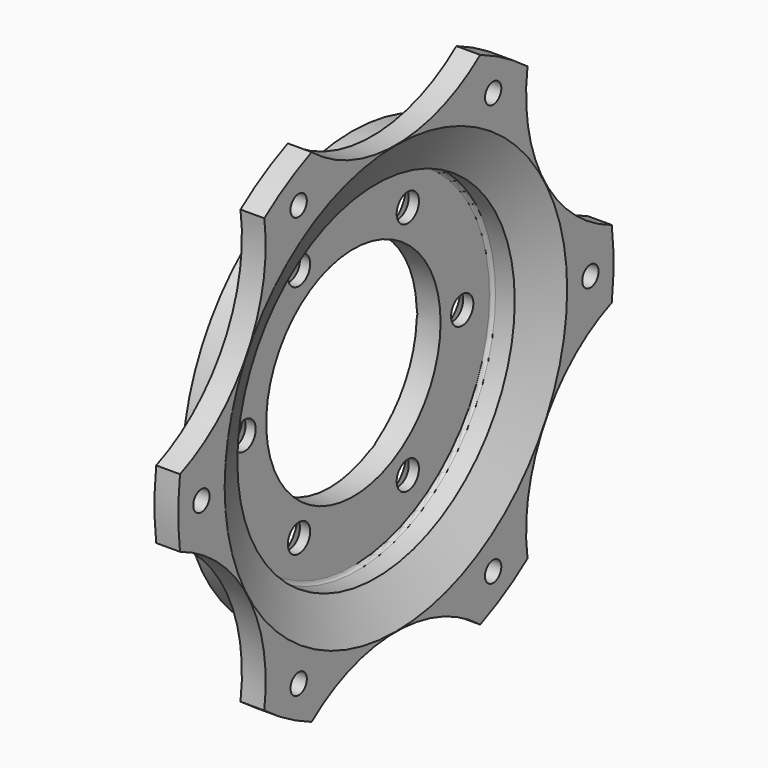
from build123d import *

# Parameters (mm, degrees)
F2_R     = 4.1
F3_DEPTH = 50
F4_R     = 3
F5_DEPTH = 50
F7_R     = 1
F8_R     = 50
F9_DEPTH = 50


# Not quite as in the source:
# - a fillet or chamfer that OpenCascade refuses, or shapes differently, is made with other operations: its cross-section is extruded or revolved along the edge and cut away or added
# - a feature names something its author has since deleted; it is built from what else it names


with BuildPart() as f1:
    # F0 (on Top) → F1 (revolve)
    with BuildSketch(Plane.XY):
        Polygon((-7, 49), (-7, 32.05), (0, 32.05), (0, 51), (6.6556592449, 51), (12.5, 62.9584203143), (12.5, 80), (5.5, 80), (5.5, 62.3), (-0.5, 62.3), align=None)
    revolve(axis=Axis((-3.5, 0, 0), (1, 0, 0)))

    # F2 (on Right) → F3 (cut, symmetric)
    with BuildSketch(Plane.YZ):
        with Locations((-40, 0)):
            Circle(F2_R)
        with Locations((-20, -34.6410161514)):
            Circle(F2_R)
        with Locations((20, -34.6410161514)):
            Circle(F2_R)
        with Locations((40, 0)):
            Circle(F2_R)
        with Locations((20, 34.6410161514)):
            Circle(F2_R)
        with Locations((-20, 34.6410161514)):
            Circle(F2_R)
    extrude(amount=F3_DEPTH, both=True, mode=Mode.SUBTRACT)

    # F4 (on face) → F5 (cut, symmetric)
    with BuildSketch(Plane(origin=(5.5, 0, 0), x_dir=(0, -1, 0), z_dir=(-1, 0, 0))):
        with Locations((35.75, 61.9208163706)):
            Circle(F4_R)
        with Locations((-35.75, 61.9208163706)):
            Circle(F4_R)
        with Locations((-71.5, 0)):
            Circle(F4_R)
        with Locations((-35.75, -61.9208163706)):
            Circle(F4_R)
        with Locations((35.75, -61.9208163706)):
            Circle(F4_R)
        with Locations((71.5, 0)):
            Circle(F4_R)
    extrude(amount=F5_DEPTH, both=True, mode=Mode.SUBTRACT)

    # F6: chamfer of 4 on 6 edges, made by hand

    # F6_s1 → F6_t2 (revolve, cut)
    with BuildSketch(Plane.XY.offset(34.6410161514)):
        Polygon((-7, 28.1), (-3, 24.1), (-7, 24.1), align=None)
    revolve(axis=Axis((-7, 20, 34.6410161514), (1, 0, 0)), mode=Mode.SUBTRACT)

    # F6_s3 → F6_t4 (revolve, cut)
    with BuildSketch(Plane.XY.offset(34.6410161514)):
        Polygon((-7, -11.9), (-3, -15.9), (-7, -15.9), align=None)
    revolve(axis=Axis((-7, -20, 34.6410161514), (1, 0, 0)), mode=Mode.SUBTRACT)

    # F6_s5 → F6_t6 (revolve, cut)
    with BuildSketch(Plane.XY):
        Polygon((-7, -31.9), (-3, -35.9), (-7, -35.9), align=None)
    revolve(axis=Axis((-7, -40, 0), (1, 0, 0)), mode=Mode.SUBTRACT)

    # F6_s7 → F6_t8 (revolve, cut)
    with BuildSketch(Plane.XY.offset(-34.6410161514)):
        Polygon((-7, -11.9), (-3, -15.9), (-7, -15.9), align=None)
    revolve(axis=Axis((-7, -20, -34.6410161514), (1, 0, 0)), mode=Mode.SUBTRACT)

    # F6_s9 → F6_t10 (revolve, cut)
    with BuildSketch(Plane.XY.offset(-34.6410161514)):
        Polygon((-7, 28.1), (-3, 24.1), (-7, 24.1), align=None)
    revolve(axis=Axis((-7, 20, -34.6410161514), (1, 0, 0)), mode=Mode.SUBTRACT)

    # F6_s11 → F6_t12 (revolve, cut)
    with BuildSketch(Plane.XY):
        Polygon((-7, 48.1), (-3, 44.1), (-7, 44.1), align=None)
    revolve(axis=Axis((-7, 40, 0), (1, 0, 0)), mode=Mode.SUBTRACT)

    # F7
    f7_edges = [f1.edges().sort_by_distance(p)[0] for p in [
        (0, -51, 0),
    ]]
    fillet(f7_edges, radius=F7_R)

    # F8 (on face) → F9 (cut, symmetric)
    with BuildSketch(Plane(origin=(5.5, 0, 0), x_dir=(0, -1, 0), z_dir=(-1, 0, 0))):
        with Locations((0, 113)):
            Circle(F8_R)
        with Locations((-97.8608706276, 56.5)):
            Circle(F8_R)
        with Locations((-97.8608706276, -56.5)):
            Circle(F8_R)
        with Locations((0, -113)):
            Circle(F8_R)
        with Locations((97.8608706276, -56.5)):
            Circle(F8_R)
        with Locations((97.8608706276, 56.5)):
            Circle(F8_R)
    extrude(amount=F9_DEPTH, both=True, mode=Mode.SUBTRACT)


solid = f1.part
